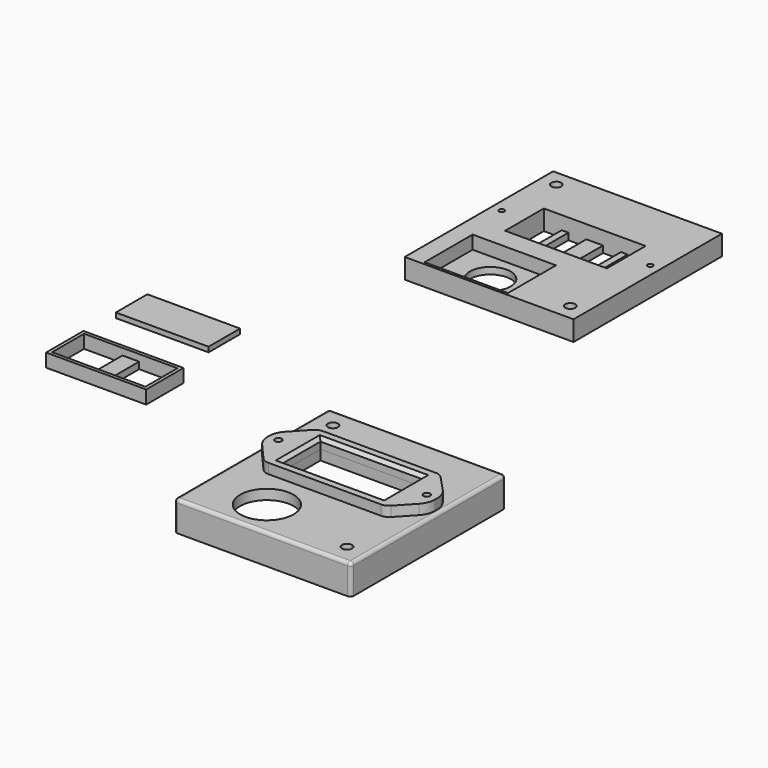
from build123d import *

# Parameters (mm, degrees)
F0_W      = 51
F0_H      = 56
F0_R      = 6.1
F0_R_2    = 1.5
F0_W_2    = 5
F0_H_2    = 14.5
F1_DEPTH  = 1
F2_W      = 30
F2_H      = 14
F5_DEPTH  = 4
F2_W_2    = 51
F2_H_2    = 56
F2_R      = 8
F2_R_2    = 1.5
F2_R_3    = 0.8
F2_W_3    = 30.5
F2_H_3    = 14.5
F6_DEPTH  = 3
F2_W_4    = 5
F2_H_4    = 2
F2_H_5    = 5
F7_DEPTH  = 2
F3_W      = 27.8
F3_H      = 11.8
F8_DEPTH  = 1.5
F2_H_6    = 1
F9_DEPTH  = 9
F10_W     = 36.5
F10_H     = 20.5
F10_W_2   = 30.5
F10_H_2   = 14.5
F10_R     = 1
F11_DEPTH = 3
F12_R     = 6
F13_R     = 3
F14_R     = 1
F15_SIZE  = 1
F18_DEPTH = 1
F19_D     = 1.4
F19_DEPTH = 1.001
F21_D     = 1.4
F16_W     = 51
F16_H     = 56
F16_W_2   = 25
F16_H_2   = 18
F16_R     = 1.5
F22_DEPTH = 5
F23_W     = 0.2
F23_H     = 55.6
F24_DEPTH = 25
F25_D     = 1.6
F25_DEPTH = 5.001
F26_D     = 1.6
F27_W     = 2
F27_H     = 14.5
F28_DEPTH = 2


# Not quite as in the source:
# - a feature names something its author has since deleted; it is built from what else it names


with BuildPart() as f1:
    # F0 (on Top) → F1 (new body)
    with BuildSketch(Plane.XY):
        Rectangle(F0_W, F0_H)
        with Locations((-7.5, -18)):
            Circle(F0_R, mode=Mode.SUBTRACT)
        with Locations((20.5, -23)):
            Circle(F0_R_2, mode=Mode.SUBTRACT)
        with Locations((-20.5, 23)):
            Circle(F0_R_2, mode=Mode.SUBTRACT)
        Polygon((-15.25, -2.75), (-15.25, 11.75), (-2.5, 11.75), (2.5, 11.75), (15.25, 11.75), (15.25, -2.75), (2.5, -2.75), (-2.5, -2.75), align=None, mode=Mode.SUBTRACT)
        with Locations((0, 4.5)):
            Rectangle(F0_W_2, F0_H_2)
    extrude(amount=F1_DEPTH)

    # F18 (add): a face of the model
    f18_faces = [f1.faces().sort_by_distance(p)[0] for p in [
        (0.3722548806, 0.1869472989, 1),
    ]]
    extrude(f18_faces, amount=F18_DEPTH)

    # F19 (through all, one way)
    with BuildSketch(Plane.XY.offset(1)):
        with Locations((-22.25, 4.75), (22.25, 4.75)):
            Circle(F19_D / 2)
    extrude(amount=-F19_DEPTH, mode=Mode.SUBTRACT)

    # F21 (through all)
    with Locations(Plane(origin=(0, 0, 1), x_dir=(1, 0, 0), z_dir=(0, 0, -1))):
        with Locations((-22.25, -4.75), (22.25, -4.75)):
            Hole(F21_D / 2)

    # F16 (on face) → F22 (join)
    with BuildSketch(Plane.XY.offset(1)):
        Rectangle(F16_W, F16_H)
        with Locations((-7.5, -18)):
            Rectangle(F16_W_2, F16_H_2, mode=Mode.SUBTRACT)
        with Locations((20.5, -23)):
            Circle(F16_R, mode=Mode.SUBTRACT)
        with Locations((-20.5, 23)):
            Circle(F16_R, mode=Mode.SUBTRACT)
        Polygon((-15.25, -2.75), (-15.25, 11.75), (-2.5, 11.75), (2.5, 11.75), (15.25, 11.75), (15.25, -2.75), (2.5, -2.75), (-2.5, -2.75), align=None, mode=Mode.SUBTRACT)
    extrude(amount=F22_DEPTH)

    # F23 (on face) → F24 (cut)
    with BuildSketch(Plane(origin=(0, 0, 0), x_dir=(1, 0, 0), z_dir=(0, 0, -1))):
        Polygon((25.5, 28), (-25.5, 28), (-25.5, 27.8), (-25.3, 27.8), (25.3, 27.8), (25.5, 27.8), align=None)
        with Locations((-25.4, 0)):
            Rectangle(F23_W, F23_H)
        with Locations((25.4, 0)):
            Rectangle(F23_W, F23_H)
        Polygon((-25.3, -27.8), (-25.5, -27.8), (-25.5, -28), (25.5, -28), (25.5, -27.8), (25.3, -27.8), align=None)
    extrude(amount=-F24_DEPTH, mode=Mode.SUBTRACT)

    # F25 (through all, one way)
    with BuildSketch(Plane(origin=(0, 0, 1), x_dir=(1, 0, 0), z_dir=(0, 0, -1))):
        with Locations((-22.25, -4.75), (22.25, -4.75)):
            Circle(F25_D / 2)
    extrude(amount=-F25_DEPTH, mode=Mode.SUBTRACT)

    # F26 (through all)
    with Locations(Plane.XY.offset(1)):
        with Locations((22.25, 4.75), (-22.25, 4.75)):
            Hole(F26_D / 2)

    # F27 (on face) → F28 (join)
    with BuildSketch(Plane(origin=(0, 0, 0), x_dir=(1, 0, 0), z_dir=(0, 0, -1))):
        with Locations((-8.875, -4.5)):
            Rectangle(F27_W, F27_H)
        with Locations((8.875, -4.5)):
            Rectangle(F27_W, F27_H)
    extrude(amount=-F28_DEPTH)


with BuildPart() as f5:
    # F2 (on Top) → F5 (new body)
    with BuildSketch(Plane.XY):
        with Locations((-48.0005137329, -108.0776734079)):
            Rectangle(F2_W, F2_H)
        Polygon((-62.0005137329, -114.0776734079), (-62.0005137329, -102.0776734079), (-50.5005137329, -102.0776734079), (-45.5005137329, -102.0776734079), (-34.0005137329, -102.0776734079), (-34.0005137329, -107.0776734079), (-34.0005137329, -109.0776734079), (-34.0005137329, -114.0776734079), (-45.5005137329, -114.0776734079), (-50.5005137329, -114.0776734079), align=None, mode=Mode.SUBTRACT)
    extrude(amount=F5_DEPTH)

    # F2 (on Top) → F7 (join)
    with BuildSketch(Plane.XY):
        with Locations((-48.0005137329, -108.0776734079)):
            Rectangle(F2_W_4, F2_H_4)
        with Locations((-48.0005137329, -104.5776734079)):
            Rectangle(F2_W_4, F2_H_5)
        with Locations((-48.0005137329, -111.5776734079)):
            Rectangle(F2_W_4, F2_H_5)
    extrude(amount=F7_DEPTH)


with BuildPart() as f6:
    # F2 (on Top) → F6 (new body)
    with BuildSketch(Plane.XY):
        with Locations((28.2103444552, -118.9687541723)):
            Rectangle(F2_W_2, F2_H_2)
        with Locations((20.7103444552, -136.9687541723)):
            Circle(F2_R, mode=Mode.SUBTRACT)
        with Locations((48.7103444552, -141.9687541723)):
            Circle(F2_R_2, mode=Mode.SUBTRACT)
        with Locations((5.9603444552, -114.2187541723)):
            Circle(F2_R_3, mode=Mode.SUBTRACT)
        with Locations((28.2103444552, -114.4687541723)):
            Rectangle(F2_W_3, F2_H_3, mode=Mode.SUBTRACT)
        with Locations((50.4603444552, -114.2187541723)):
            Circle(F2_R_3, mode=Mode.SUBTRACT)
        with Locations((7.7103444552, -95.9687541723)):
            Circle(F2_R_2, mode=Mode.SUBTRACT)
    extrude(amount=-F6_DEPTH)

    # F2 (on Top) → F9 (join)
    with BuildSketch(Plane.XY):
        Polygon((2.7103444552, -146.9687541723), (2.7103444552, -90.9687541723), (2.7103444552, -89.9687541723), (1.7103444552, -89.9687541723), (1.7103444552, -147.9687541723), (2.7103444552, -147.9687541723), align=None)
        with Locations((28.2103444552, -90.4687541723)):
            Rectangle(F2_W_2, F2_H_6)
        with Locations((28.2103444552, -147.4687541723)):
            Rectangle(F2_W_2, F2_H_6)
        Polygon((53.7103444552, -89.9687541723), (53.7103444552, -90.9687541723), (53.7103444552, -146.9687541723), (53.7103444552, -147.9687541723), (54.7103444552, -147.9687541723), (54.7103444552, -89.9687541723), align=None)
    extrude(amount=-F9_DEPTH)

    # F14
    f14_edges = [f6.edges().sort_by_distance(p)[0] for p in [
        (1.710344, -118.968754, 0),
        (28.210344, -89.968754, 0),
        (28.210344, -147.968754, 0),
        (54.710344, -118.968754, 0),
        (54.710344, -147.968754, -4.5),
        (1.710344, -147.968754, -4.5),
        (1.710344, -89.968754, -4.5),
        (54.710344, -89.968754, -4.5),
    ]]
    fillet(f14_edges, radius=F14_R)


with BuildPart() as f8:
    # F3 (on Top) → F8 (new body)
    with BuildSketch(Plane.XY):
        with Locations((-52.0366017878, -79.3675661445)):
            Rectangle(F3_W, F3_H)
    extrude(amount=F8_DEPTH)


with BuildPart() as f11:
    # F10 (on face) → F11 (new body)
    with BuildSketch(Plane.XY):
        with Locations((28.2103444552, -114.4687541723)):
            Rectangle(F10_W, F10_H)
        with Locations((28.2103444552, -114.4687541723)):
            Rectangle(F10_W_2, F10_H_2, mode=Mode.SUBTRACT)
        Polygon((9.9603444552, -124.7187541723), (9.9603444552, -104.2187541723), (2.9603444552, -111.7187541723), (2.9603444552, -116.7187541723), align=None)
        with Locations((5.9603444552, -114.2187541723)):
            Circle(F10_R, mode=Mode.SUBTRACT)
        Polygon((53.4603444552, -111.7187541723), (46.4603444552, -104.2187541723), (46.4603444552, -124.7187541723), (53.4603444552, -117.2187541723), align=None)
        with Locations((50.4603444552, -114.2187541723)):
            Circle(F10_R, mode=Mode.SUBTRACT)
    extrude(amount=F11_DEPTH)

    # F12
    f12_edges = [f11.edges().sort_by_distance(p)[0] for p in [
        (2.960344, -111.718754, 1.5),
        (2.960344, -116.718754, 1.5),
        (53.460344, -117.218754, 1.5),
        (53.460344, -111.718754, 1.5),
    ]]
    fillet(f12_edges, radius=F12_R)

    # F13
    f13_edges = [f11.edges().sort_by_distance(p)[0] for p in [
        (9.960344, -104.218754, 1.5),
        (9.960344, -124.718754, 1.5),
        (46.460344, -124.718754, 1.5),
        (46.460344, -104.218754, 1.5),
    ]]
    fillet(f13_edges, radius=F13_R)

    # F15
    f15_edges = [f11.edges().sort_by_distance(p)[0] for p in [
        (12.960344, -114.468754, 3),
        (28.210344, -107.218754, 3),
        (43.460344, -114.468754, 3),
        (28.210344, -121.718754, 3),
    ]]
    chamfer(f15_edges, length=F15_SIZE)


solid = Compound([f1.part, f5.part, f6.part, f8.part, f11.part])
